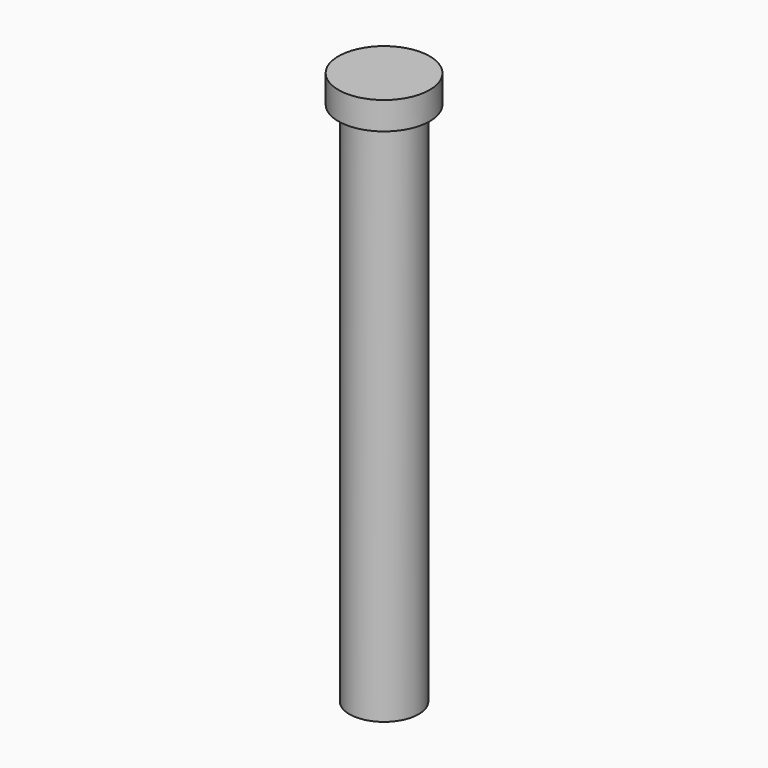
from build123d import *

# Parameters (mm, degrees)
F1_R     = 7.9375
F2_DEPTH = 60.325
F3_R     = 10.4775
F4_DEPTH = 6.35


# Not quite as in the source:
# - a variable given as a bare number and used for a length is read in inches; the dataset says mm whatever the document's units were


with BuildPart() as f2:
    # F1 (on Top) → F2 (new body, symmetric)
    with BuildSketch(Plane.XY):
        Circle(F1_R)
    extrude(amount=F2_DEPTH, both=True)

    # F3 (on face) → F4 (join)
    with BuildSketch(Plane.XY.offset(60.325)):
        Circle(F3_R)
    extrude(amount=F4_DEPTH)


solid = f2.part
